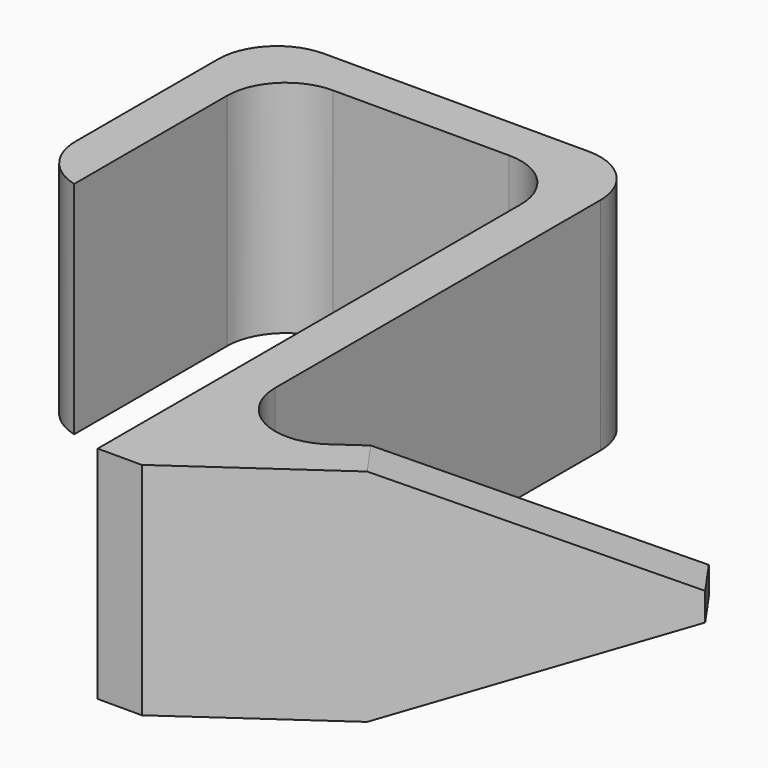
from build123d import *

# Parameters (mm, degrees)
F1_DEPTH     = 19.05
F2_T1_DEPTH  = 19.05
F2_T3_DEPTH  = 19.05
F2_T5_DEPTH  = 19.05
F2_T7_DEPTH  = 44.45
F2_T9_DEPTH  = 44.45
F2_T11_DEPTH = 43.6434442484
F3_SIZE2     = 8.3203595553
F3_SIZE      = 22.86
F3_2_SIZE2   = 8.3203595553
F3_2_SIZE    = 22.86


# Not quite as in the source:
# - a fillet or chamfer that OpenCascade refuses, or shapes differently, is made with other operations: its cross-section is extruded or revolved along the edge and cut away or added


with BuildPart() as f1:
    # F0 (on Top) → F1 (new body)
    with BuildSketch(Plane.XY):
        Polygon((-33.02, 29.6357684863), (-33.02, 4.2357684863), (-29.21, 4.2357684863), (-29.21, 25.8257684863), (-3.81, 25.8257684863), (-3.81, -24.9742315137), (0, -24.9742315137), (31.2096928874, -3.1209692887), (29.0243666649, 0), (0, -20.3230803305), (0, 29.6357684863), align=None)
    extrude(amount=F1_DEPTH)

    # F2: fillet of radius 5.08 on 6 edges, made by hand

    # F2_s2 → F2_t1 (join)
    with BuildSketch(Plane.XY):
        with BuildLine():
            ThreePointArc((7.9937682967, -14.7257835105), (2.7343170448, -15.0705061581), (0, -10.5644911255))
            Line((0, -10.5644911255), (0, -20.3230803305))
            Line((0, -20.3230803305), (7.9937682967, -14.7257835105))
        make_face()
    extrude(amount=F2_T1_DEPTH)

    # F2_s4 → F2_t3 (join)
    with BuildSketch(Plane.XY):
        with BuildLine():
            ThreePointArc((-29.21, 20.7457684863), (-27.7221024484, 24.3378709347), (-24.13, 25.8257684863))
            Line((-24.13, 25.8257684863), (-29.21, 25.8257684863))
            Line((-29.21, 25.8257684863), (-29.21, 20.7457684863))
        make_face()
    extrude(amount=F2_T3_DEPTH)

    # F2_s6 → F2_t5 (join)
    with BuildSketch(Plane.XY):
        with BuildLine():
            ThreePointArc((-8.89, 25.8257684863), (-5.2978975516, 24.3378709347), (-3.81, 20.7457684863))
            Line((-3.81, 20.7457684863), (-3.81, 25.8257684863))
            Line((-3.81, 25.8257684863), (-8.89, 25.8257684863))
        make_face()
    extrude(amount=F2_T5_DEPTH)

    # F2_s8 → F2_t7 (cut)
    with BuildSketch(Plane.XY.offset(-12.7)):
        with BuildLine():
            ThreePointArc((0, 24.5557684863), (-1.4878975516, 28.1478709347), (-5.08, 29.6357684863))
            Line((-5.08, 29.6357684863), (0, 29.6357684863))
            Line((0, 29.6357684863), (0, 24.5557684863))
        make_face()
    extrude(amount=F2_T7_DEPTH, mode=Mode.SUBTRACT)

    # F2_s10 → F2_t9 (cut)
    with BuildSketch(Plane.XY.offset(-12.7)):
        with BuildLine():
            ThreePointArc((-33.02, 24.5557684863), (-31.5321024484, 28.1478709347), (-27.94, 29.6357684863))
            Line((-27.94, 29.6357684863), (-33.02, 29.6357684863))
            Line((-33.02, 29.6357684863), (-33.02, 24.5557684863))
        make_face()
    extrude(amount=F2_T9_DEPTH, mode=Mode.SUBTRACT)

    # F2_s12 → F2_t11 (cut)
    with BuildSketch(Plane.XY.offset(-12.2967221242)):
        with BuildLine():
            ThreePointArc((-29.21, 4.2357684863), (-31.9560926284, 6.0436053626), (-33.02, 9.154457336))
            Line((-33.02, 9.154457336), (-33.02, 4.2357684863))
            Line((-33.02, 4.2357684863), (-29.21, 4.2357684863))
        make_face()
    extrude(amount=F2_T11_DEPTH, mode=Mode.SUBTRACT)

    # F3
    f3_edges = [f1.edges().sort_by_distance(p)[0] for p in [
        (30.11703, -1.560485, 19.05),
    ]]
    f3_side = f1.faces().sort_by_distance((-2.966928, -2.114232, 19.05))[0]
    chamfer(f3_edges, length=F3_SIZE, length2=F3_SIZE2, reference=f3_side)

    # F3#2
    f3_2_edges = [f1.edges().sort_by_distance(p)[0] for p in [
        (30.11703, -1.560485, 0),
    ]]
    f3_2_side = f1.faces().sort_by_distance((-2.966928, -2.114232, 0))[0]
    chamfer(f3_2_edges, length=F3_2_SIZE, length2=F3_2_SIZE2, reference=f3_2_side)


solid = f1.part
